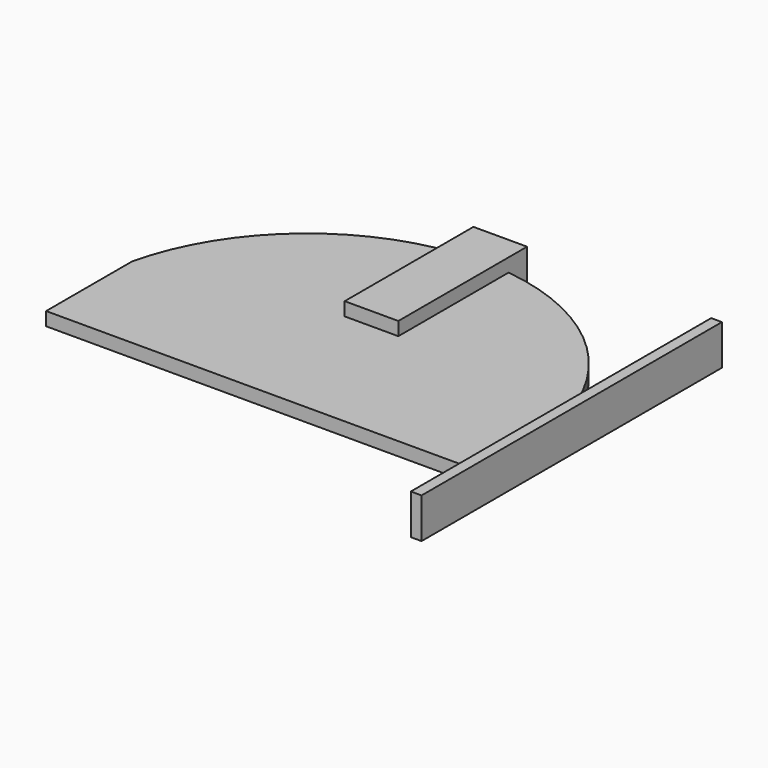
from build123d import *

# Parameters (mm, degrees)
F1_DEPTH = 1.5875
F2_DEPTH = 1.5875
F3_DEPTH = 4.7625
F4_DEPTH = 4.7625
F5_W     = 19.05
F5_H     = 3.175
F5_W_2   = 25.4
F5_W_3   = 44.45
F6_DEPTH = 2.54


with BuildPart() as f1:
    # F0 (on Top) → F1 (new body)
    with BuildSketch(Plane.XY):
        with BuildLine():
            Line((-50.8, 0), (0, 0))
            Line((0, 0), (50.8, 0))
            Line((50.8, 0), (50.8, 25.4))
            ThreePointArc((50.8, 25.4), (34.8924839126, 52.4357961473), (6.35, 65.4477119742))
            Line((6.35, 65.4477119742), (6.35, 32.8159203153))
            Line((6.35, 32.8159203153), (0, 32.8159203153))
            Line((0, 32.8159203153), (-6.35, 32.8159203153))
            Line((-6.35, 32.8159203153), (-6.35, 65.4477119742))
            ThreePointArc((-6.35, 65.4477119742), (-34.8924839126, 52.4357961473), (-50.8, 25.4))
            Line((-50.8, 25.4), (-50.8, 0))
        make_face()
    extrude(amount=F1_DEPTH)

    # F2 (add): a face of the model
    f2_faces = [f1.faces().sort_by_distance(p)[0] for p in [
        (0, 27.1005445022, 0),
    ]]
    extrude(f2_faces, amount=F2_DEPTH)

    # F0 (on Top) → F3 (join)
    with BuildSketch(Plane.XY):
        with BuildLine():
            ThreePointArc((6.35, 65.4477119742), (0, 65.8359203153), (-6.35, 65.4477119742))
            Line((-6.35, 65.4477119742), (-6.35, 32.8159203153))
            Line((-6.35, 32.8159203153), (0, 32.8159203153))
            Line((0, 32.8159203153), (6.35, 32.8159203153))
            Line((6.35, 32.8159203153), (6.35, 65.4477119742))
        make_face()
        with BuildLine():
            Line((-6.35, 70.9159203153), (-6.35, 65.4477119742))
            ThreePointArc((-6.35, 65.4477119742), (0, 65.8359203153), (6.35, 65.4477119742))
            Line((6.35, 65.4477119742), (6.35, 70.9159203153))
            Line((6.35, 70.9159203153), (0, 70.9159203153))
            Line((0, 70.9159203153), (-6.35, 70.9159203153))
        make_face()
    extrude(amount=F3_DEPTH)

    # F0 (on Top) → F4 (join)
    with BuildSketch(Plane.XY):
        with BuildLine():
            ThreePointArc((6.35, 65.4477119742), (0, 65.8359203153), (-6.35, 65.4477119742))
            Line((-6.35, 65.4477119742), (-6.35, 32.8159203153))
            Line((-6.35, 32.8159203153), (0, 32.8159203153))
            Line((0, 32.8159203153), (6.35, 32.8159203153))
            Line((6.35, 32.8159203153), (6.35, 65.4477119742))
        make_face()
        with BuildLine():
            Line((-6.35, 70.9159203153), (-6.35, 65.4477119742))
            ThreePointArc((-6.35, 65.4477119742), (0, 65.8359203153), (6.35, 65.4477119742))
            Line((6.35, 65.4477119742), (6.35, 70.9159203153))
            Line((6.35, 70.9159203153), (0, 70.9159203153))
            Line((0, 70.9159203153), (-6.35, 70.9159203153))
        make_face()
    extrude(amount=-F4_DEPTH)

    # F5 (on face) → F6 (join)
    with BuildSketch(Plane.YZ.offset(50.8)):
        with Locations((-9.525, 0)):
            Rectangle(F5_W, F5_H)
        Polygon((-19.05, 1.5875), (0, 1.5875), (25.4, 1.5875), (69.85, 1.5875), (69.85, 4.7625), (-19.05, 4.7625), align=None)
        with Locations((12.7, 0)):
            Rectangle(F5_W_2, F5_H)
        with Locations((47.625, 0)):
            Rectangle(F5_W_3, F5_H)
        Polygon((25.4, -1.5875), (0, -1.5875), (-19.05, -1.5875), (-19.05, -4.7625), (69.85, -4.7625), (69.85, -1.5875), align=None)
    extrude(amount=F6_DEPTH)


solid = f1.part
